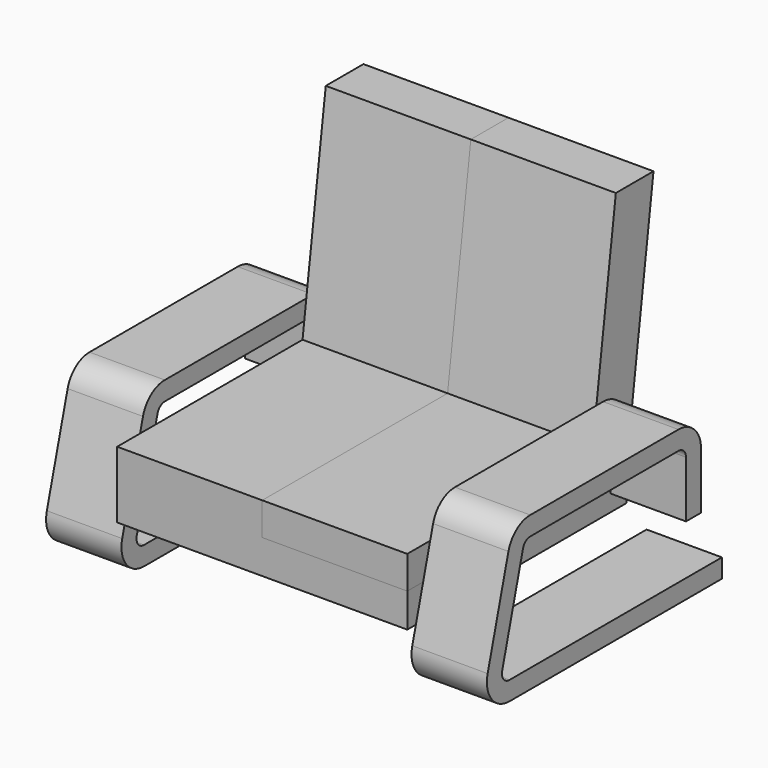
from build123d import *

# Parameters (mm, degrees)
F1_W       = 1170
F1_H       = 50
F3_W       = 770
F3_H       = 900
F4_DEPTH   = 600
F6_DEPTH   = 385
F7_DEPTH   = 385
F7_FACE_W  = 385
F7_FACE_H  = 728.0723833729
F7_FACE1_W = 385
F7_FACE1_H = 728.0723833729
F8_DEPTH   = 90


# Not quite as in the source:
# - an extrude ends at something that could not be found from the text; its depth is read off the source's solid


with BuildPart() as f2:
    # F2: sweep along a path in F0
    with BuildLine(Plane.YZ) as f2_path:
        Line((65.9058558057, 70.2815868228), (-638.9328755523, 70.2815868228))
        ThreePointArc((-638.9328755523, 70.2815868228), (-678.6005425668, 89.8435153723), (-687.2291668667, 133.2225390779))
        Line((-687.2291668667, 133.2225390779), (-618.2610394219, 390.6150948048))
        ThreePointArc((-618.2610394219, 390.6150948048), (-600.4028195579, 417.3418095643), (-569.9647481074, 427.6741425497))
        Line((-569.9647481074, 427.6741425497), (-78.3310975064, 427.6741425497))
        ThreePointArc((-78.3310975064, 427.6741425497), (-42.9757584471, 413.029481609), (-28.3310975064, 377.6741425497))
        Line((-28.3310975064, 377.6741425497), (-28.3310975064, 227.6741425497))
    # F1 (on Front) → F2 (sweep)
    with BuildSketch(Plane.XZ):
        with Locations((0, 70.2815868228)):
            Rectangle(F1_W, F1_H)
    sweep(path=f2_path.line)

    # F3 (on Top) → F4 (cut)
    with BuildSketch(Plane.XY):
        with Locations((0, -311.2359523773)):
            Rectangle(F3_W, F3_H)
    extrude(amount=F4_DEPTH, mode=Mode.SUBTRACT)


with BuildPart() as f6:
    # F5 (on Right) → F6 (new body, through all)
    with BuildSketch(Plane.YZ):
        Polygon((-728.0723833729, 361.0842398319), (-728.0723833729, 274.0944385529), (0, 274.0944385529), (88.9778784892, 923.0227374731), (-36.0221215108, 923.0227374731), (-113.0723833729, 361.0842398319), align=None)
    extrude(amount=F6_DEPTH)


with BuildPart() as f7:
    # F7 (new, through all): a face of the model
    f7_faces = [f6.part.faces().sort_by_distance(p)[0] for p in [
        (0, -420.5723833729, 350.6502613598),
    ]]
    extrude(f7_faces, amount=F7_DEPTH)

    # F7_face (on face) + F7_face1 (on face) → F8 (join)
    with BuildSketch(Plane(origin=(192.5, -364.0361916864, 274.0944385529), x_dir=(1, 0, 0), z_dir=(0, 0, -1))):
        Rectangle(F7_FACE_W, F7_FACE_H)
    with BuildSketch(Plane(origin=(-192.5, -364.0361916864, 274.0944385529), x_dir=(1, 0, 0), z_dir=(0, 0, -1))):
        Rectangle(F7_FACE1_W, F7_FACE1_H)
    extrude(amount=F8_DEPTH)


solid = Compound([f2.part, f6.part, f7.part])
